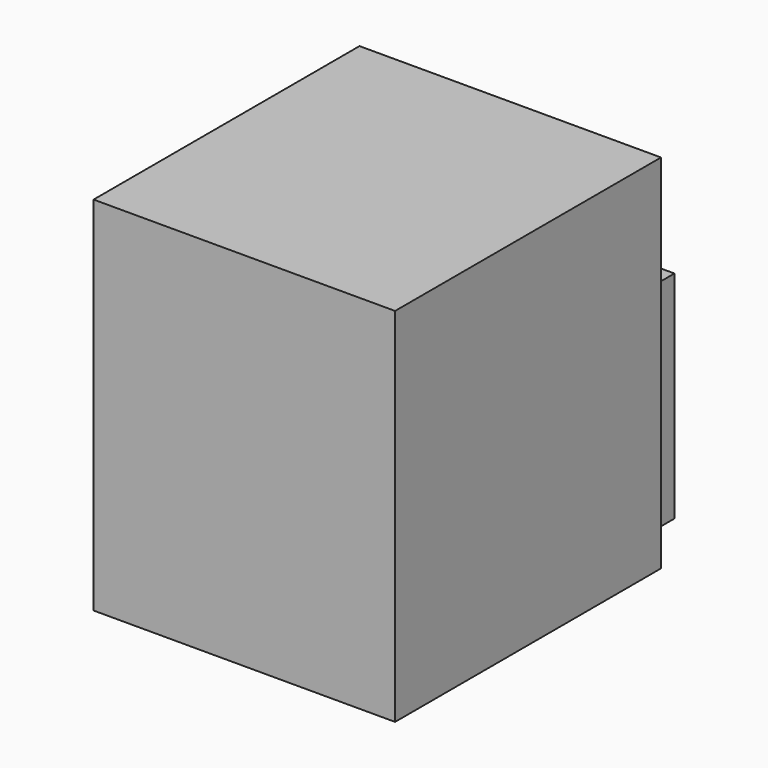
from build123d import *

# Parameters (mm, degrees)
F0_W      = 105.8345548809
F0_H      = 111.5989610553
F1_DEPTH  = 127
F2_W      = 105.8345548809
F2_H      = 127
F2_W_2    = 22.996397689
F2_H_2    = 22.2293362021
F3_DEPTH  = 5.08
F4_W      = 26.9106691703
F4_H      = 50.3869839013
F5_DEPTH  = 5.08
F7_DEPTH  = 25.4
F8_W      = 22.5071115419
F8_H      = 21.3920027018
F9_DEPTH  = 5.08
F10_W     = 22.0178281888
F10_H     = 21.4731246233
F11_DEPTH = 5.08
F12_W     = 10.2898292243
F12_H     = 61.8074573576
F13_DEPTH = 5.08


with BuildPart() as f1:
    # F0 (on Top) → F1 (new body)
    with BuildSketch(Plane.XY):
        with Locations((0.5764421076, -0.230576843)):
            Rectangle(F0_W, F0_H)
    extrude(amount=F1_DEPTH)

    # F2 (on face) → F3 (join)
    with BuildSketch(Plane(origin=(0, 55.5689036846, 0), x_dir=(-1, 0, 0), z_dir=(0, 1, 0))):
        with Locations((-0.5764421076, 63.5)):
            Rectangle(F2_W, F2_H)
        with Locations((-31.7689729854, 99.5473898947)):
            Rectangle(F2_W_2, F2_H_2, mode=Mode.SUBTRACT)
    extrude(amount=F3_DEPTH)

    # F4 (on face) → F5 (join)
    with BuildSketch(Plane(origin=(0, 60.6489036846, 0), x_dir=(-1, 0, 0), z_dir=(0, 1, 0))):
        with Locations((-1.4360728674, 25.1934919506)):
            Rectangle(F4_W, F4_H)
    extrude(amount=F5_DEPTH)

    # F6 (on face) → F7 (join)
    with BuildSketch(Plane(origin=(0, 60.6489036846, 0), x_dir=(-1, 0, 0), z_dir=(0, 1, 0))):
        Polygon((-37.8878116608, 0), (-29.5699629933, 0), (-29.5699629933, 55.8542273939), (22.2942437977, 55.8542273939), (22.2942437977, 0), (32.1800485253, 0), (32.1800485253, 75.7494047284), (-37.8878116608, 75.7494047284), align=None)
        Polygon((-29.5699629933, 55.8542273939), (-29.5699629933, 0), (-14.8914074525, 0), (-14.8914074525, 50.3869839013), (12.0192617178, 50.3869839013), (12.0192617178, 0), (22.2942437977, 0), (22.2942437977, 55.8542273939), align=None)
    extrude(amount=F7_DEPTH)

    # F8 (on face) → F9 (cut)
    with BuildSketch(Plane(origin=(0, 60.6489036846, 0), x_dir=(-1, 0, 0), z_dir=(0, 1, 0))):
        with Locations((-3.1485739164, 100.074402988)):
            Rectangle(F8_W, F8_H)
    extrude(amount=-F9_DEPTH, mode=Mode.SUBTRACT)

    # F10 (on face) → F11 (cut)
    with BuildSketch(Plane(origin=(0, 60.6489036846, 0), x_dir=(-1, 0, 0), z_dir=(0, 1, 0))):
        with Locations((24.006747175, 100.1149639487)):
            Rectangle(F10_W, F10_H)
    extrude(amount=-F11_DEPTH, mode=Mode.SUBTRACT)

    # F12 (on face) → F13 (cut)
    with BuildSketch(Plane(origin=(0, 86.0489036846, 0), x_dir=(-1, 0, 0), z_dir=(0, 1, 0))):
        with Locations((-27.1603707224, 30.9037286788)):
            Rectangle(F12_W, F12_H)
    extrude(amount=-F13_DEPTH, mode=Mode.SUBTRACT)


solid = f1.part
